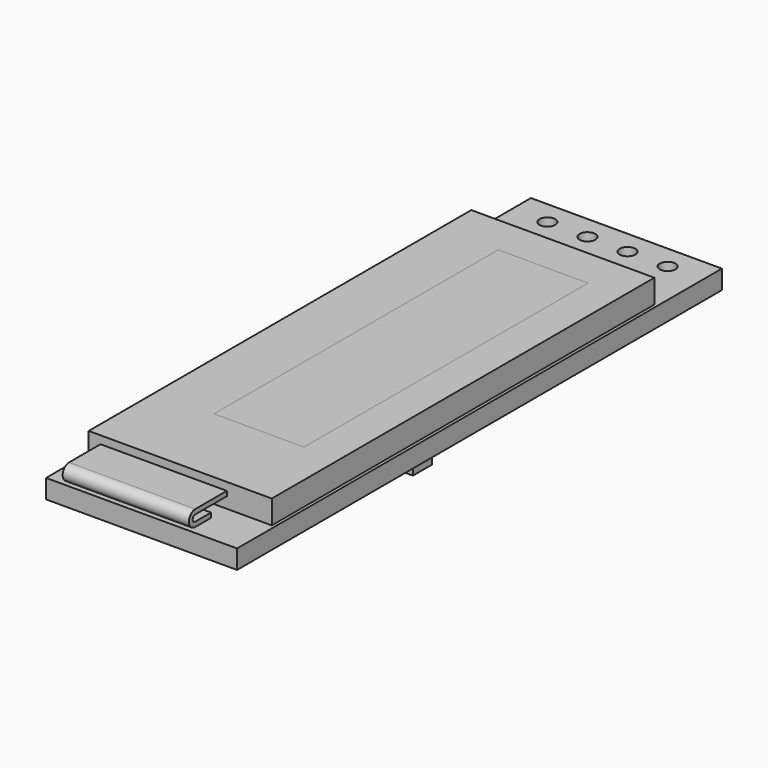
from build123d import *

# Parameters (mm, degrees)
F0_W          = 12.1
F0_H          = 38.4
F0_R          = 0.5
F1_DEPTH      = 1.2
F2_W          = 11.6
F2_H          = 30.3
F2_W_2        = 5.7
F2_H_2        = 22.5
F3_DEPTH      = 1.5
F4_DEPTH      = 1.5
F6_DEPTH      = 3
F6_DEPTH_BACK = 5
F7_W          = 0.762
F7_H          = 1.524
F7_W_2        = 3
F7_H_2        = 1.65
F8_DEPTH      = 0.9


with BuildPart() as f1:
    # F0 (on Top) → F1 (new body)
    with BuildSketch(Plane.XY):
        with Locations((0, 19.2)):
            Rectangle(F0_W, F0_H)
        with Locations((-3.81, 36.9)):
            Circle(F0_R, mode=Mode.SUBTRACT)
        with Locations((-1.27, 36.9)):
            Circle(F0_R, mode=Mode.SUBTRACT)
        with Locations((1.27, 36.9)):
            Circle(F0_R, mode=Mode.SUBTRACT)
        with Locations((3.81, 36.9)):
            Circle(F0_R, mode=Mode.SUBTRACT)
    extrude(amount=-F1_DEPTH)

    # F7 (on face) → F8 (join)
    with BuildSketch(Plane(origin=(0, 0, -1.2), x_dir=(1, 0, 0), z_dir=(0, 0, -1))):
        with Locations((5.069, -15.438)):
            Rectangle(F7_W, F7_H)
        with Locations((3.6492857143, -15.438)):
            Rectangle(F7_W, F7_H)
        with Locations((2.2295714286, -15.438)):
            Rectangle(F7_W, F7_H)
        with Locations((0.8098571429, -15.438)):
            Rectangle(F7_W, F7_H)
        with Locations((-0.6098571429, -15.438)):
            Rectangle(F7_W, F7_H)
        with Locations((-2.0295714286, -15.438)):
            Rectangle(F7_W, F7_H)
        with Locations((-1.25, -28.875)):
            Rectangle(F7_W_2, F7_H_2)
        with Locations((-3.4492857143, -15.438)):
            Rectangle(F7_W, F7_H)
        with Locations((-4.869, -15.438)):
            Rectangle(F7_W, F7_H)
        with Locations((2.769, -22.138)):
            Rectangle(F7_W, F7_H)
        with Locations((1.3095, -22.138)):
            Rectangle(F7_W, F7_H)
        with Locations((-0.15, -22.138)):
            Rectangle(F7_W, F7_H)
        with Locations((-1.6095, -22.138)):
            Rectangle(F7_W, F7_H)
        with Locations((-3.069, -22.138)):
            Rectangle(F7_W, F7_H)
    extrude(amount=F8_DEPTH)


with BuildPart() as f3:
    # F2 (on Top) → F3 (new body)
    with BuildSketch(Plane.XY):
        with Locations((0.05, 18.15)):
            Rectangle(F2_W, F2_H)
        with Locations((0.8, 19.55)):
            Rectangle(F2_W_2, F2_H_2, mode=Mode.SUBTRACT)
    extrude(amount=F3_DEPTH)

    # F5 (on Right) → F6 (join, two sides)
    with BuildSketch(Plane.YZ) as f6_sk:
        with BuildLine():
            Line((3, 1), (0.5, 1))
            ThreePointArc((0.5, 1), (0, 0.5), (0.5, 0))
            Line((0.5, 0), (1.7500170507, 0))
            Line((1.7500170507, 0), (1.7500170507, 0.3))
            Line((1.7500170507, 0.3), (0.5, 0.3))
            ThreePointArc((0.5, 0.3), (0.3, 0.5), (0.5, 0.7))
            Line((0.5, 0.7), (3, 0.7))
            Line((3, 0.7), (3, 1))
        make_face()
    extrude(amount=F6_DEPTH)
    extrude(f6_sk.sketch, amount=-F6_DEPTH_BACK)


with BuildPart() as f4:
    # F2 (on Top) → F4 (new body, through all)
    with BuildSketch(Plane.XY):
        with Locations((0.8, 19.55)):
            Rectangle(F2_W_2, F2_H_2)
    extrude(amount=F4_DEPTH)


solid = Compound([f1.part, f3.part, f4.part])
